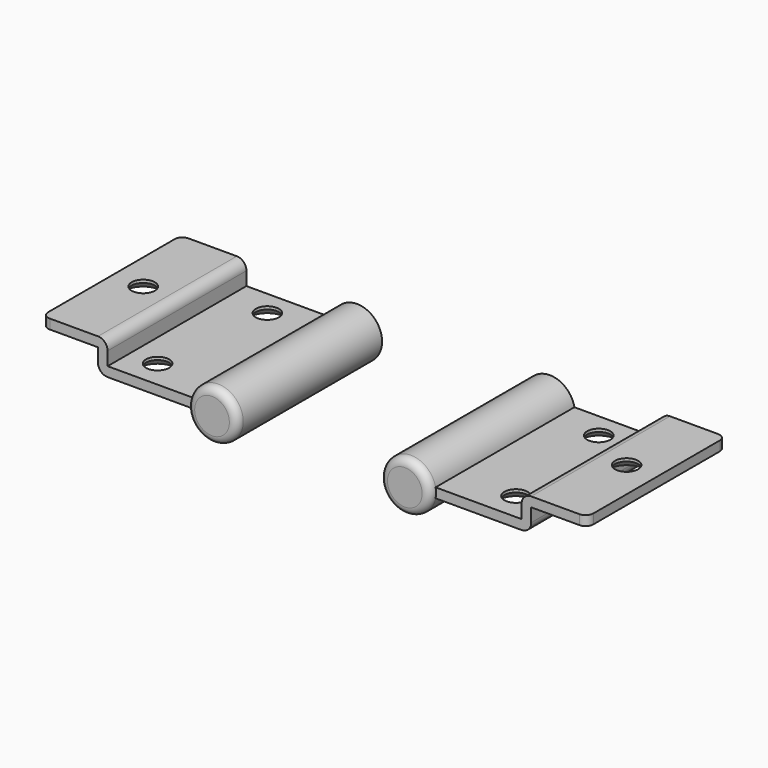
from build123d import *

# Parameters (mm, degrees)
F0_R            = 4
F1_DEPTH        = 45
F2_R            = 2
F3_R            = 2.5
F5_D            = 6
F5_CSINK_D      = 9.5
F5_CSINK_ANGLE  = 90
F6_R            = 6.5
F7_DEPTH        = 2
F8_R            = 1.99999
F10_D           = 6
F10_CSINK_D     = 9.5
F10_CSINK_ANGLE = 90


# Not quite as in the source:
# - a fillet or chamfer is up to 0.001 mm smaller than in the source, because OpenCascade refuses the exact size
# - a feature names something its author has since deleted; it is built from what else it names


with BuildPart() as f1:
    # F0 (on Front) → F1 (new body)
    with BuildSketch(Plane.XZ):
        with BuildLine():
            Line((28.6786754111, 1.25), (6.3786754111, 1.25))
            ThreePointArc((6.3786754111, 1.25), (-6.5, 0), (6.3786754111, -1.25))
            Line((6.3786754111, -1.25), (31.1786754111, -1.25))
            Line((31.1786754111, -1.25), (31.1786754111, 4.75))
            Line((31.1786754111, 4.75), (45.6786754111, 4.75))
            Line((45.6786754111, 4.75), (45.6786754111, 7.25))
            Line((45.6786754111, 7.25), (28.6786754111, 7.25))
            Line((28.6786754111, 7.25), (28.6786754111, 1.25))
        make_face()
        Circle(F0_R, mode=Mode.SUBTRACT)
    extrude(amount=F1_DEPTH)

    # F2
    f2_edges = [f1.edges().sort_by_distance(p)[0] for p in [
        (45.678675, -45, 6),
        (45.678675, 0, 6),
    ]]
    fillet(f2_edges, radius=F2_R)

    # F3
    f3_edges = [f1.edges().sort_by_distance(p)[0] for p in [
        (31.178675, -22.5, -1.25),
        (28.678675, -22.5, 7.25),
    ]]
    fillet(f3_edges, radius=F3_R)

    # F5 (through all)
    with Locations(Plane(origin=(0, 0, -1.25), x_dir=(1, 0, 0), z_dir=(0, 0, -1))):
        with Locations((17.9786754111, 6.6), (21.4786754111, 37.8)):
            CounterSinkHole(F5_D / 2, F5_CSINK_D / 2, counter_sink_angle=F5_CSINK_ANGLE)

    # F6 (on face) → F7 (join)
    with BuildSketch(Plane.XZ.offset(45)):
        Circle(F6_R)
    extrude(amount=F7_DEPTH)

    # F8 (radius 2 in the source; OpenCascade refuses exactly that, so slightly less here)
    f8_edges = [f1.edges().sort_by_distance(p)[0] for p in [
        (-6.5, -47, 0),
    ]]
    fillet(f8_edges, radius=F8_R)

    # F10 (through all)
    with Locations(Plane(origin=(0, 0, 4.75), x_dir=(1, 0, 0), z_dir=(0, 0, -1))):
        with Locations((37.6786754111, 22.2)):
            CounterSinkHole(F10_D / 2, F10_CSINK_D / 2, counter_sink_angle=F10_CSINK_ANGLE)


with BuildPart() as f12_1:
    # F12: instance of F1
    add(f1.part.mirror(Plane.YZ.offset(-25)))


solid = Compound([f1.part, f12_1.part])
